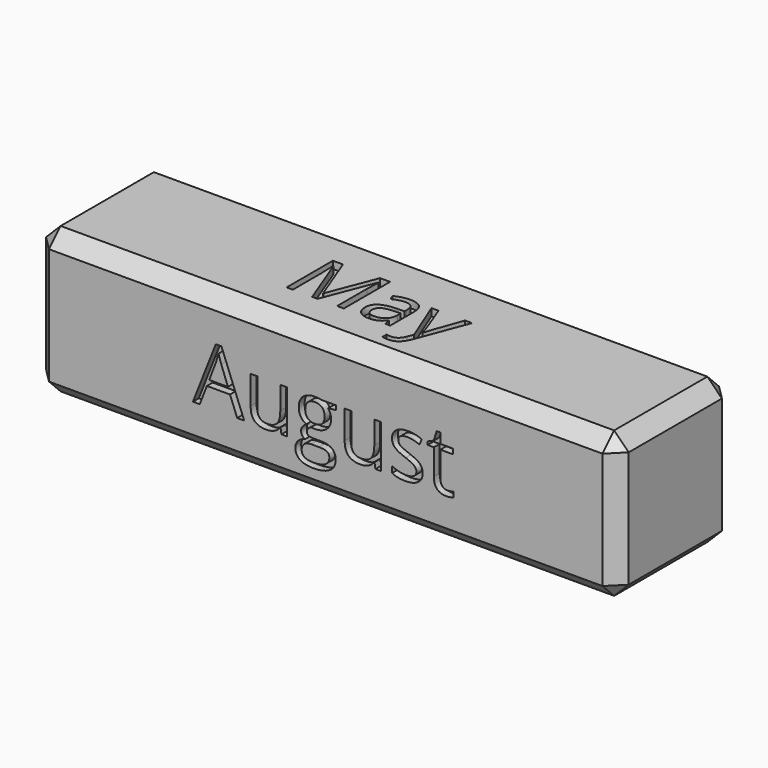
from build123d import *

# Parameters (mm, degrees)
F0_W          = 101.6
F0_H          = 25.4
F1_DEPTH      = 12.7
F1_DEPTH_BACK = 12.7
F2_SIZE       = 2.54
F3_TEXT_SIZE  = 14.1111111111
F4_DEPTH      = 1.27
F5_TEXT_SIZE  = 14.1111111111
F6_DEPTH      = 1.27
F7_TEXT_SIZE  = 14.1111111111
F8_DEPTH      = 1.27
F9_TEXT_SIZE  = 14.1111111111
F10_DEPTH     = 1.27


# Not quite as in the source:
# - Text() gives the source's letters only with a copy of the font that has no kerning and outlines rounded to 1/6400 em; it was checked with that copy


with BuildPart() as f1:
    # F0 (on Top) → F1 (new body, two sides)
    with BuildSketch(Plane.XY) as f1_sk:
        Rectangle(F0_W, F0_H)
    extrude(amount=F1_DEPTH)
    extrude(f1_sk.sketch, amount=-F1_DEPTH_BACK)

    # F2
    f2_edges = [f1.edges().sort_by_distance(p)[0] for p in [
        (50.8, 0, 12.7),
        (0, 12.7, 12.7),
        (-50.8, 0, 12.7),
        (0, -12.7, 12.7),
        (-50.8, -12.7, 0),
        (50.8, -12.7, 0),
        (0, -12.7, -12.7),
        (-50.8, 0, -12.7),
        (-50.8, 12.7, 0),
        (50.8, 0, -12.7),
        (0, 12.7, -12.7),
        (50.8, 12.7, 0),
    ]]
    chamfer(f2_edges, length=F2_SIZE)

    # F3 (on face) → F4 (cut)
    with BuildSketch(Plane.XY.offset(12.7)):
        with Locations((-14.2996267361, -5.08)):
            Text('May', F3_TEXT_SIZE, font='Open Sans', text_align=(TextAlign.LEFT, TextAlign.BOTTOM))
    extrude(amount=-F4_DEPTH, mode=Mode.SUBTRACT)

    # F5 (on face) → F6 (cut)
    with BuildSketch(Plane(origin=(0, 12.7, 0), x_dir=(-1, 0, 0), z_dir=(0, 1, 0))):
        with Locations(Location((15.1429861111, 5.08), (0, 0, -180))):
            Text('June', F5_TEXT_SIZE, font='Open Sans', text_align=(TextAlign.LEFT, TextAlign.BOTTOM))
    extrude(amount=-F6_DEPTH, mode=Mode.SUBTRACT)

    # F7 (on face) → F8 (cut)
    with BuildSketch(Plane(origin=(0, 0, -12.7), x_dir=(1, 0, 0), z_dir=(0, 0, -1))):
        with Locations((-12.5566840278, -5.08)):
            Text('July', F7_TEXT_SIZE, font='Open Sans', text_align=(TextAlign.LEFT, TextAlign.BOTTOM))
    extrude(amount=-F8_DEPTH, mode=Mode.SUBTRACT)

    # F9 (on face) → F10 (cut)
    with BuildSketch(Plane.XZ.offset(12.7)):
        with Locations((-23.1565538194, -5.08)):
            Text('August', F9_TEXT_SIZE, font='Open Sans', text_align=(TextAlign.LEFT, TextAlign.BOTTOM))
    extrude(amount=-F10_DEPTH, mode=Mode.SUBTRACT)


solid = f1.part
